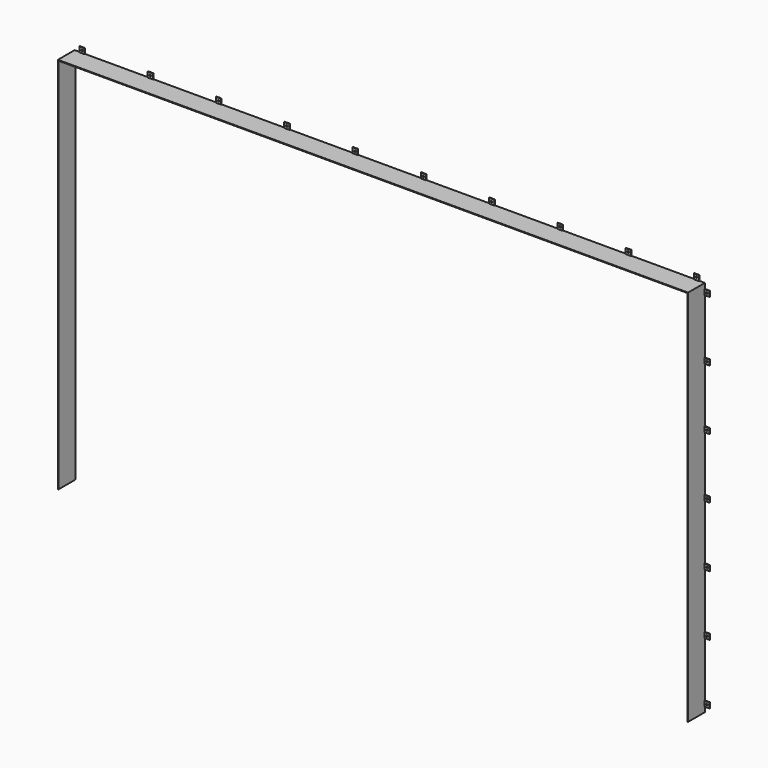
from build123d import *

# Parameters (mm, degrees)
F1_DEPTH = 101.6
F0_W     = 25.4
F0_H     = 25.4
F0_R     = 3.81
F2_DEPTH = 3.175


# Not quite as in the source:
# - a feature names something its author has since deleted; it is built from what else it names


with BuildPart() as f1:
    # F0 (on Front) → F1 (new body)
    with BuildSketch(Plane.XZ):
        Polygon((0, 25.4), (0, 0), (3.175, 0), (3.175, 1828.8), (3051.175, 1828.8), (3051.175, 0), (3054.35, 0), (3054.35, 25.4), (3054.35, 50.8), (3054.35, 318.0291666667), (3054.35, 343.4291666667), (3054.35, 610.6583333333), (3054.35, 636.0583333333), (3054.35, 903.2875), (3054.35, 928.6875), (3054.35, 1195.9166666667), (3054.35, 1221.3166666667), (3054.35, 1488.5458333333), (3054.35, 1513.9458333333), (3054.35, 1781.175), (3054.35, 1806.575), (3054.35, 1831.975), (3028.95, 1831.975), (3003.55, 1831.975), (2698.0444444444, 1831.975), (2672.6444444444, 1831.975), (2367.1388888889, 1831.975), (2341.7388888889, 1831.975), (2036.2333333333, 1831.975), (2010.8333333333, 1831.975), (1705.3277777778, 1831.975), (1679.9277777778, 1831.975), (1374.4222222222, 1831.975), (1349.0222222222, 1831.975), (1043.5166666667, 1831.975), (1018.1166666667, 1831.975), (712.6111111111, 1831.975), (687.2111111111, 1831.975), (381.7055555556, 1831.975), (356.3055555556, 1831.975), (50.8, 1831.975), (25.4, 1831.975), (0, 1831.975), (0, 1806.575), (0, 1781.175), (0, 1513.9458333333), (0, 1488.5458333333), (0, 1221.3166666667), (0, 1195.9166666667), (0, 928.6875), (0, 903.2875), (0, 636.0583333333), (0, 610.6583333333), (0, 343.4291666667), (0, 318.0291666667), (0, 50.8), align=None)
    extrude(amount=F1_DEPTH)

    # F0 (on Front) → F2 (join)
    with BuildSketch(Plane.XZ):
        with Locations((-12.7, 38.1)):
            Rectangle(F0_W, F0_H)
        with Locations((-12.7, 38.1)):
            Circle(F0_R, mode=Mode.SUBTRACT)
        with Locations((-12.7, 330.7291666667)):
            Rectangle(F0_W, F0_H)
        with Locations((-12.7, 330.7291666667)):
            Circle(F0_R, mode=Mode.SUBTRACT)
        with Locations((-12.7, 623.3583333333)):
            Rectangle(F0_W, F0_H)
        with Locations((-12.7, 623.3583333333)):
            Circle(F0_R, mode=Mode.SUBTRACT)
        with Locations((3067.05, 38.1)):
            Rectangle(F0_W, F0_H)
        with Locations((3067.05, 38.1)):
            Circle(F0_R, mode=Mode.SUBTRACT)
        with Locations((-12.7, 915.9875)):
            Rectangle(F0_W, F0_H)
        with Locations((-12.7, 915.9875)):
            Circle(F0_R, mode=Mode.SUBTRACT)
        with Locations((3067.05, 330.7291666667)):
            Rectangle(F0_W, F0_H)
        with Locations((3067.05, 330.7291666667)):
            Circle(F0_R, mode=Mode.SUBTRACT)
        with Locations((-12.7, 1208.6166666667)):
            Rectangle(F0_W, F0_H)
        with Locations((-12.7, 1208.6166666667)):
            Circle(F0_R, mode=Mode.SUBTRACT)
        with Locations((3067.05, 623.3583333333)):
            Rectangle(F0_W, F0_H)
        with Locations((3067.05, 623.3583333333)):
            Circle(F0_R, mode=Mode.SUBTRACT)
        with Locations((-12.7, 1501.2458333333)):
            Rectangle(F0_W, F0_H)
        with Locations((-12.7, 1501.2458333333)):
            Circle(F0_R, mode=Mode.SUBTRACT)
        with Locations((3067.05, 915.9875)):
            Rectangle(F0_W, F0_H)
        with Locations((3067.05, 915.9875)):
            Circle(F0_R, mode=Mode.SUBTRACT)
        with Locations((-12.7, 1793.875)):
            Rectangle(F0_W, F0_H)
        with Locations((-12.7, 1793.875)):
            Circle(F0_R, mode=Mode.SUBTRACT)
        with Locations((3067.05, 1208.6166666667)):
            Rectangle(F0_W, F0_H)
        with Locations((3067.05, 1208.6166666667)):
            Circle(F0_R, mode=Mode.SUBTRACT)
        with Locations((38.1, 1844.675)):
            Rectangle(F0_W, F0_H)
        with Locations((38.1, 1844.675)):
            Circle(F0_R, mode=Mode.SUBTRACT)
        with Locations((3067.05, 1501.2458333333)):
            Rectangle(F0_W, F0_H)
        with Locations((3067.05, 1501.2458333333)):
            Circle(F0_R, mode=Mode.SUBTRACT)
        with Locations((369.0055555556, 1844.675)):
            Rectangle(F0_W, F0_H)
        with Locations((369.0055555556, 1844.675)):
            Circle(F0_R, mode=Mode.SUBTRACT)
        with Locations((3067.05, 1793.875)):
            Rectangle(F0_W, F0_H)
        with Locations((3067.05, 1793.875)):
            Circle(F0_R, mode=Mode.SUBTRACT)
        with Locations((699.9111111111, 1844.675)):
            Rectangle(F0_W, F0_H)
        with Locations((699.9111111111, 1844.675)):
            Circle(F0_R, mode=Mode.SUBTRACT)
        with Locations((3016.25, 1844.675)):
            Rectangle(F0_W, F0_H)
        with Locations((3016.25, 1844.675)):
            Circle(F0_R, mode=Mode.SUBTRACT)
        with Locations((1030.8166666667, 1844.675)):
            Rectangle(F0_W, F0_H)
        with Locations((1030.8166666667, 1844.675)):
            Circle(F0_R, mode=Mode.SUBTRACT)
        with Locations((2685.3444444444, 1844.675)):
            Rectangle(F0_W, F0_H)
        with Locations((2685.3444444444, 1844.675)):
            Circle(F0_R, mode=Mode.SUBTRACT)
        with Locations((1361.7222222222, 1844.675)):
            Rectangle(F0_W, F0_H)
        with Locations((1361.7222222222, 1844.675)):
            Circle(F0_R, mode=Mode.SUBTRACT)
        with Locations((2354.4388888889, 1844.675)):
            Rectangle(F0_W, F0_H)
        with Locations((2354.4388888889, 1844.675)):
            Circle(F0_R, mode=Mode.SUBTRACT)
        with Locations((1692.6277777778, 1844.675)):
            Rectangle(F0_W, F0_H)
        with Locations((1692.6277777778, 1844.675)):
            Circle(F0_R, mode=Mode.SUBTRACT)
        with Locations((2023.5333333333, 1844.675)):
            Rectangle(F0_W, F0_H)
        with Locations((2023.5333333333, 1844.675)):
            Circle(F0_R, mode=Mode.SUBTRACT)
    extrude(amount=F2_DEPTH)


solid = f1.part
